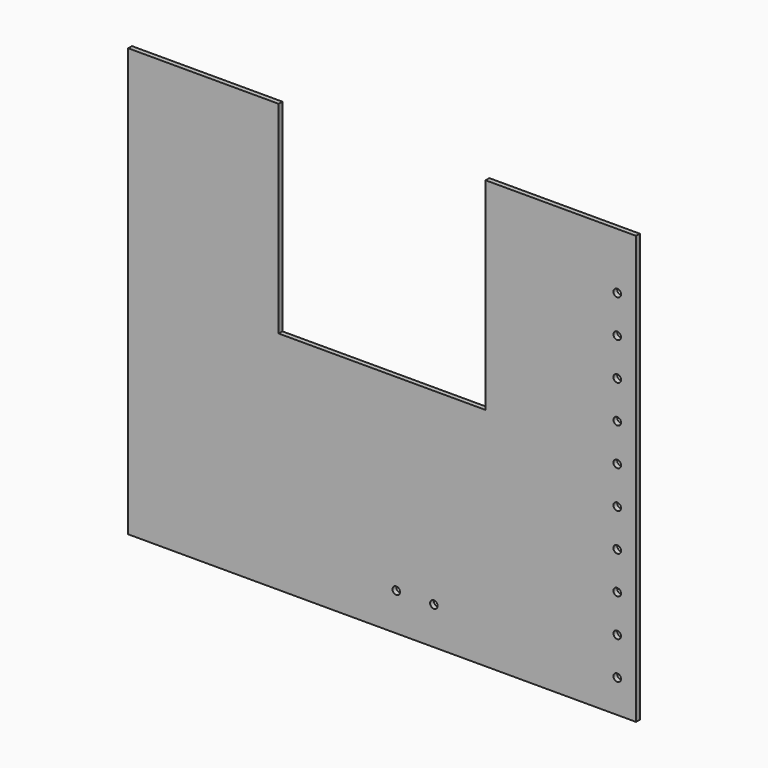
from build123d import *

# Parameters (mm, degrees)
F0_R     = 2.5527
F1_DEPTH = 3.175


with BuildPart() as f1:
    # F0 (on Front) → F1 (new body)
    with BuildSketch(Plane.XZ):
        Polygon((0, 288.925), (0, 0), (342.9, 0), (342.9, 288.925), (241.3, 288.925), (241.3, 152.4), (101.6, 152.4), (101.6, 288.925), align=None)
        with Locations((181.0013651848, 25.4)):
            Circle(F0_R, mode=Mode.SUBTRACT)
        with Locations((206.4013651848, 25.4)):
            Circle(F0_R, mode=Mode.SUBTRACT)
        with Locations((330.2, 22.225)):
            Circle(F0_R, mode=Mode.SUBTRACT)
        with Locations((330.2, 47.625)):
            Circle(F0_R, mode=Mode.SUBTRACT)
        with Locations((330.2, 73.025)):
            Circle(F0_R, mode=Mode.SUBTRACT)
        with Locations((330.2, 98.425)):
            Circle(F0_R, mode=Mode.SUBTRACT)
        with Locations((330.2, 123.825)):
            Circle(F0_R, mode=Mode.SUBTRACT)
        with Locations((330.2, 149.225)):
            Circle(F0_R, mode=Mode.SUBTRACT)
        with Locations((330.2, 174.625)):
            Circle(F0_R, mode=Mode.SUBTRACT)
        with Locations((330.2, 200.025)):
            Circle(F0_R, mode=Mode.SUBTRACT)
        with Locations((330.2, 225.425)):
            Circle(F0_R, mode=Mode.SUBTRACT)
        with Locations((330.2, 250.825)):
            Circle(F0_R, mode=Mode.SUBTRACT)
    extrude(amount=F1_DEPTH)


solid = f1.part
